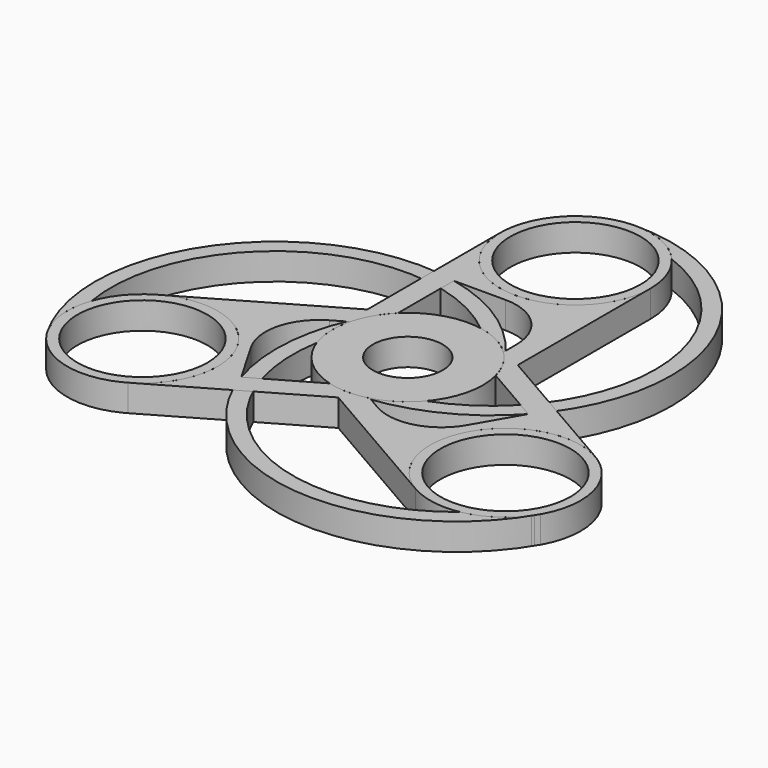
from build123d import *

# Parameters (mm, degrees)
F0_R      = 14
F1_DEPTH  = 5
F2_R      = 6.5
F3_DEPTH  = 5
F4_R      = 14
F5_DEPTH  = 5
F6_R      = 12.1
F7_DEPTH  = 5
F9_DEPTH  = 5
F11_DEPTH = 5
F12_W     = 19.6309629187
F12_H     = 13.4950243425
F13_DEPTH = 25
F14_R     = 10


# Not quite as in the source:
# - a feature names something its author has since deleted; it is built from what else it names


with BuildPart() as f1:
    # F0 (on Top) → F1 (new body)
    with BuildSketch(Plane.XY):
        Circle(F0_R)
    extrude(amount=F1_DEPTH)

    # F2 (on face) → F3 (cut)
    with BuildSketch(Plane.XY.offset(5)):
        Circle(F2_R)
    extrude(amount=-F3_DEPTH, mode=Mode.SUBTRACT)


with BuildPart() as f5:
    # F4 (on Top) → F5 (new body)
    with BuildSketch(Plane.XY):
        with Locations((0, 39)):
            Circle(F4_R)
    extrude(amount=F5_DEPTH)


with BuildPart() as f5b:
    # F4 (on Top) → F5, piece 2 (new body)
    with BuildSketch(Plane.XY):
        with Locations((-33.7749907476, -19.5)):
            Circle(F4_R)
    extrude(amount=F5_DEPTH)


with BuildPart() as f5c:
    # F4 (on Top) → F5, piece 3 (new body)
    with BuildSketch(Plane.XY):
        with Locations((33.7749907476, -19.5)):
            Circle(F4_R)
    extrude(amount=F5_DEPTH)


with BuildPart() as f7_tool:
    # F6 (on face) → F7 (new body)
    with BuildSketch(Plane.XY.offset(5)):
        with Locations((0, 39)):
            Circle(F6_R)
        with Locations((-33.7749907476, -19.5)):
            Circle(F6_R)
        with Locations((33.7749907476, -19.5)):
            Circle(F6_R)
    extrude(amount=-F7_DEPTH)


with BuildPart() as f5_1:
    add(f5.part)

    # F7: cut by f7_tool
    add(f7_tool.part, mode=Mode.SUBTRACT)


with BuildPart() as f5b_1:
    add(f5b.part)

    # F7: cut by f7_tool
    add(f7_tool.part, mode=Mode.SUBTRACT)


with BuildPart() as f5c_1:
    add(f5c.part)

    # F7: cut by f7_tool
    add(f7_tool.part, mode=Mode.SUBTRACT)


with BuildPart() as f9:
    # F8 (on face) → F9 (new body)
    with BuildSketch(Plane.XY.offset(5)):
        with BuildLine():
            ThreePointArc((10.6587742004, -9.0769230769), (5.8703950856, -12.709778186), (0, -14))
            ThreePointArc((0, -14), (33.5, 19.5), (0, 53))
            ThreePointArc((0, 53), (5.8703950856, 51.709778186), (10.6587742004, 48.0769230769))
            ThreePointArc((10.6587742004, 48.0769230769), (30.5, 19.5), (10.6587742004, -9.0769230769))
        make_face()
    extrude(amount=-F9_DEPTH)


with BuildPart() as f9b:
    # F8 (on face) → F9, piece 2 (new body)
    with BuildSketch(Plane.XY.offset(5)):
        with BuildLine():
            ThreePointArc((2.5314588726, 13.7692307692), (8.0717932428, 11.4388003674), (12.124355653, 7))
            ThreePointArc((12.124355653, 7), (-33.6374953738, 19.2618510268), (-45.8993464006, -26.5))
            ThreePointArc((-45.8993464006, -26.5), (-47.717179076, -20.7709778186), (-46.9652238206, -14.8076923077))
            ThreePointArc((-46.9652238206, -14.8076923077), (-32.1374953738, 16.6637748154), (2.5314588726, 13.7692307692))
        make_face()
    extrude(amount=-F9_DEPTH)


with BuildPart() as f9c:
    # F8 (on face) → F9, piece 3 (new body)
    with BuildSketch(Plane.XY.offset(5)):
        with BuildLine():
            ThreePointArc((-13.190233073, -4.6923076923), (-13.9421883284, 1.2709778186), (-12.124355653, 7))
            ThreePointArc((-12.124355653, 7), (0.1374953738, -38.7618510268), (45.8993464006, -26.5))
            ThreePointArc((45.8993464006, -26.5), (41.8467839904, -30.9388003674), (36.3064496202, -33.2692307692))
            ThreePointArc((36.3064496202, -33.2692307692), (1.6374953738, -36.1637748154), (-13.190233073, -4.6923076923))
        make_face()
    extrude(amount=-F9_DEPTH)


with BuildPart() as f11:
    # F10 (on face) → F11 (new body)
    with BuildSketch(Plane.XY.offset(5)):
        with BuildLine():
            ThreePointArc((-7, -12.124355653), (-12.124355653, -7), (-14, 0))
            Line((-14, 0), (-14, 8.0829037687))
            Line((-14, 8.0829037687), (-40.7749907476, -7.375644347))
            ThreePointArc((-40.7749907476, -7.375644347), (-21.6506350946, -12.5), (-26.7749907476, -31.624355653))
            Line((-26.7749907476, -31.624355653), (0, -16.1658075373))
            Line((0, -16.1658075373), (-7, -12.124355653))
        make_face()
        with BuildLine():
            Line((-14, 8.0829037687), (-14, 0))
            ThreePointArc((-14, 0), (-12.124355653, 7), (-7, 12.124355653))
            Line((-7, 12.124355653), (-14, 8.0829037687))
        make_face()
        with BuildLine():
            Line((-14, 39), (-14, 8.0829037687))
            Line((-14, 8.0829037687), (-7, 12.124355653))
            ThreePointArc((-7, 12.124355653), (0, 14), (7, 12.124355653))
            Line((7, 12.124355653), (14, 8.0829037687))
            Line((14, 8.0829037687), (14, 39))
            ThreePointArc((14, 39), (0, 25), (-14, 39))
        make_face()
        with BuildLine():
            ThreePointArc((7, -12.124355653), (0, -14), (-7, -12.124355653))
            Line((-7, -12.124355653), (0, -16.1658075373))
            Line((0, -16.1658075373), (7, -12.124355653))
        make_face()
        with BuildLine():
            Line((14, 8.0829037687), (7, 12.124355653))
            ThreePointArc((7, 12.124355653), (12.124355653, 7), (14, 0))
            Line((14, 0), (14, 8.0829037687))
        make_face()
        with BuildLine():
            ThreePointArc((14, 0), (12.124355653, -7), (7, -12.124355653))
            Line((7, -12.124355653), (0, -16.1658075373))
            Line((0, -16.1658075373), (26.7749907476, -31.624355653))
            ThreePointArc((26.7749907476, -31.624355653), (21.6506350946, -12.5), (40.7749907476, -7.375644347))
            Line((40.7749907476, -7.375644347), (14, 8.0829037687))
            Line((14, 8.0829037687), (14, 0))
        make_face()
    extrude(amount=-F11_DEPTH)

    # F12 (on face) → F13 (cut)
    with BuildSketch(Plane.XY.offset(5)):
        with Locations((0, 16.2475121713)):
            Rectangle(F12_W, F12_H)
        Polygon((-3.3195006063, -13.2504562942), (-13.1349820656, 3.7504562942), (-24.822015971, -2.9970558771), (-15.0065345116, -19.9979684655), align=None)
        Polygon((13.1349820656, 3.7504562942), (3.3195006063, -13.2504562942), (15.0065345116, -19.9979684655), (24.822015971, -2.9970558771), align=None)
    extrude(amount=-F13_DEPTH, mode=Mode.SUBTRACT)

    # F14
    f14_edges = [f11.edges().sort_by_distance(p)[0] for p in [
        (9.815481, 22.995024, 2.5),
        (15.006535, -19.997968, 2.5),
        (-24.822016, -2.997056, 2.5),
    ]]
    fillet(f14_edges, radius=F14_R)


solid = Compound([f1.part, f5_1.part, f5b_1.part, f5c_1.part, f9.part, f9b.part, f9c.part, f11.part])
